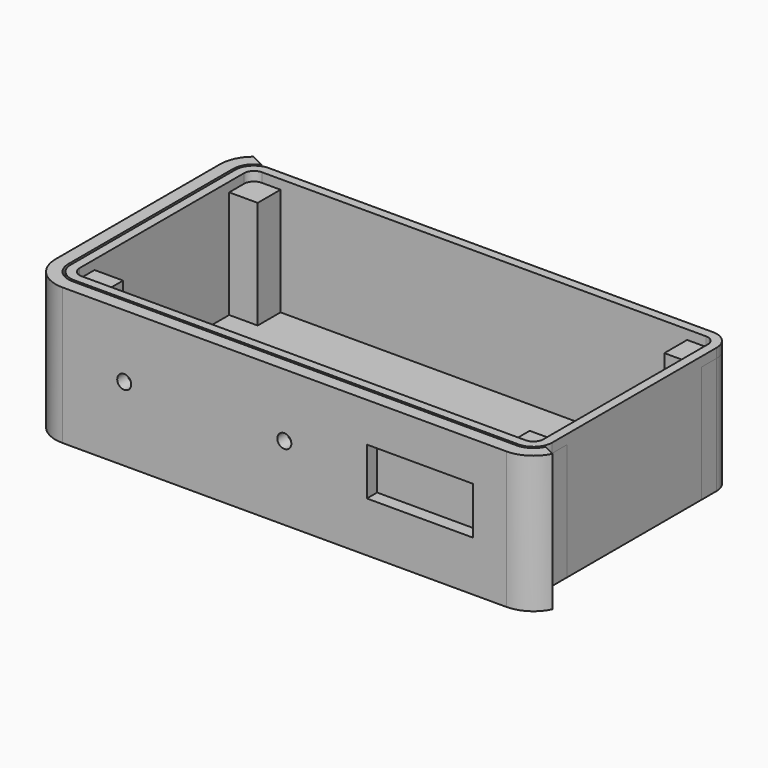
from build123d import *

# Parameters (mm, degrees)
F1_DEPTH  = 27
F2_T      = -1.9
F4_DEPTH  = 25
F9_DEPTH  = 27
F10_T     = -2.75
F6_R      = 1.5
F6_W      = 22.75
F6_H      = 10.15
F11_DEPTH = 25
F5_R      = 1.5
F12_DEPTH = 25
F14_DEPTH = 30
F15_DEPTH = 5
F16_DEPTH = 2.3
F17_DEPTH = 2.7


with BuildPart() as f1:
    # F0 (on Top) → F1 (new body)
    with BuildSketch(Plane.XY):
        Polygon((43.5, 18), (43.5, 26), (-43.5, 26), (-43.5, 18), (-51.5, 18), (-51.5, -18), (-43.5, -18), (-43.5, -26), (43.5, -26), (43.5, -18), (51.5, -18), (51.5, 18), align=None)
        with BuildLine():
            Line((-43.5, 18), (-43.5, 26))
            Line((-43.5, 26), (-47.5, 26))
            ThreePointArc((-47.5, 26), (-50.3284271247, 24.8284271247), (-51.5, 22))
            Line((-51.5, 22), (-51.5, 18))
            Line((-51.5, 18), (-43.5, 18))
        make_face()
        with BuildLine():
            ThreePointArc((51.5, 22), (50.3284271247, 24.8284271247), (47.5, 26))
            Line((47.5, 26), (43.5, 26))
            Line((43.5, 26), (43.5, 18))
            Line((43.5, 18), (51.5, 18))
            Line((51.5, 18), (51.5, 22))
        make_face()
        with BuildLine():
            Line((51.5, -22), (51.5, -18))
            Line((51.5, -18), (43.5, -18))
            Line((43.5, -18), (43.5, -26))
            Line((43.5, -26), (47.5, -26))
            ThreePointArc((47.5, -26), (50.3284271247, -24.8284271247), (51.5, -22))
        make_face()
        with BuildLine():
            Line((-43.5, -18), (-51.5, -18))
            Line((-51.5, -18), (-51.5, -22))
            ThreePointArc((-51.5, -22), (-50.3284271247, -24.8284271247), (-47.5, -26))
            Line((-47.5, -26), (-43.5, -26))
            Line((-43.5, -26), (-43.5, -18))
        make_face()
    extrude(amount=F1_DEPTH)

    # F2
    f2_openings = [f1.faces().sort_by_distance(p)[0] for p in [
        (0, 0, 27),
    ]]
    offset(amount=F2_T, openings=f2_openings)


with BuildPart() as f4:
    # F3 (on face) → F4 (new body)
    with BuildSketch(Plane.XY):
        with BuildLine():
            Line((-43.5, 18), (-43.5, 26))
            Line((-43.5, 26), (-47.5, 26))
            ThreePointArc((-47.5, 26), (-50.3284271247, 24.8284271247), (-51.5, 22))
            Line((-51.5, 22), (-51.5, 18))
            Line((-51.5, 18), (-43.5, 18))
        make_face()
    extrude(amount=F4_DEPTH)


with BuildPart() as f4b:
    # F0 (on Top) → F4, piece 2 (new body)
    with BuildSketch(Plane.XY):
        with BuildLine():
            Line((-43.5, -18), (-51.5, -18))
            Line((-51.5, -18), (-51.5, -22))
            ThreePointArc((-51.5, -22), (-50.3284271247, -24.8284271247), (-47.5, -26))
            Line((-47.5, -26), (-43.5, -26))
            Line((-43.5, -26), (-43.5, -18))
        make_face()
    extrude(amount=F4_DEPTH)


with BuildPart() as f4c:
    # F0 (on Top) → F4, piece 3 (new body)
    with BuildSketch(Plane.XY):
        with BuildLine():
            Line((51.5, -22), (51.5, -18))
            Line((51.5, -18), (43.5, -18))
            Line((43.5, -18), (43.5, -26))
            Line((43.5, -26), (47.5, -26))
            ThreePointArc((47.5, -26), (50.3284271247, -24.8284271247), (51.5, -22))
        make_face()
    extrude(amount=F4_DEPTH)


with BuildPart() as f4d:
    # F0 (on Top) → F4, piece 4 (new body)
    with BuildSketch(Plane.XY):
        with BuildLine():
            ThreePointArc((51.5, 22), (50.3284271247, 24.8284271247), (47.5, 26))
            Line((47.5, 26), (43.5, 26))
            Line((43.5, 26), (43.5, 18))
            Line((43.5, 18), (51.5, 18))
            Line((51.5, 18), (51.5, 22))
        make_face()
    extrude(amount=F4_DEPTH)


with BuildPart() as f9:
    # F8 (on Top) → F9 (new body)
    with BuildSketch(Plane.XY):
        with BuildLine():
            Line((47.5, 29.25), (-47.5, 29.25))
            ThreePointArc((-47.5, 29.25), (-52.6265241636, 27.1265241636), (-54.75, 22))
            Line((-54.75, 22), (-54.75, -22))
            ThreePointArc((-54.75, -22), (-52.6265241636, -27.1265241636), (-47.5, -29.25))
            Line((-47.5, -29.25), (47.5, -29.25))
            ThreePointArc((47.5, -29.25), (52.6265241636, -27.1265241636), (54.75, -22))
            Line((54.75, -22), (54.75, 22))
            ThreePointArc((54.75, 22), (52.6265241636, 27.1265241636), (47.5, 29.25))
        make_face()
    extrude(amount=F9_DEPTH)

    # F10
    f10_openings = [f9.faces().sort_by_distance(p)[0] for p in [
        (0, 0, 27),
    ]]
    offset(amount=F10_T, openings=f10_openings)

    # F6 (on face) → F11 (cut)
    with BuildSketch(Plane.XZ.offset(26)):
        with Locations((-34.2500010431, 13.5)):
            Circle(F6_R)
        with Locations((0, 13.5)):
            Circle(F6_R)
        with Locations((29.0283542126, 13.5)):
            Rectangle(F6_W, F6_H)
    extrude(amount=F11_DEPTH, mode=Mode.SUBTRACT)

    # F5 (on face) → F12 (cut)
    with BuildSketch(Plane(origin=(-51.5, 0, 0), x_dir=(0, -1, 0), z_dir=(-1, 0, 0))):
        with Locations((-10.7654500753, 13.5)):
            Circle(F5_R)
    extrude(amount=F12_DEPTH, mode=Mode.SUBTRACT)

    # F13 (on Top) → F14 (cut)
    with BuildSketch(Plane.XY):
        Polygon((65.3300657868, 29.3469112366), (-55.5969104171, 29.3469112366), (62.0856769383, -29.0519669652), align=None)
    extrude(amount=F14_DEPTH, mode=Mode.SUBTRACT)

    # F15 (add): a face of the model
    f15_faces = [f9.faces().sort_by_distance(p)[0] for p in [
        (-15.8065422029, -8.455255524, 2.75),
    ]]
    extrude(f15_faces, amount=-F15_DEPTH)

    # F16 (add): a face of the model
    f16_faces = [f9.faces().sort_by_distance(p)[0] for p in [
        (-51.1894899225, 25.7891492293, 0),
    ]]
    extrude(f16_faces, amount=F16_DEPTH)

    # F17 (cut): a face of the model
    f17_faces = [f9.faces().sort_by_distance(p)[0] for p in [
        (-15.8065422029, -8.455255524, 2.75),
    ]]
    extrude(f17_faces, amount=-F17_DEPTH, mode=Mode.SUBTRACT)


solid = Compound([f1.part, f4.part, f4b.part, f4c.part, f4d.part, f9.part])
